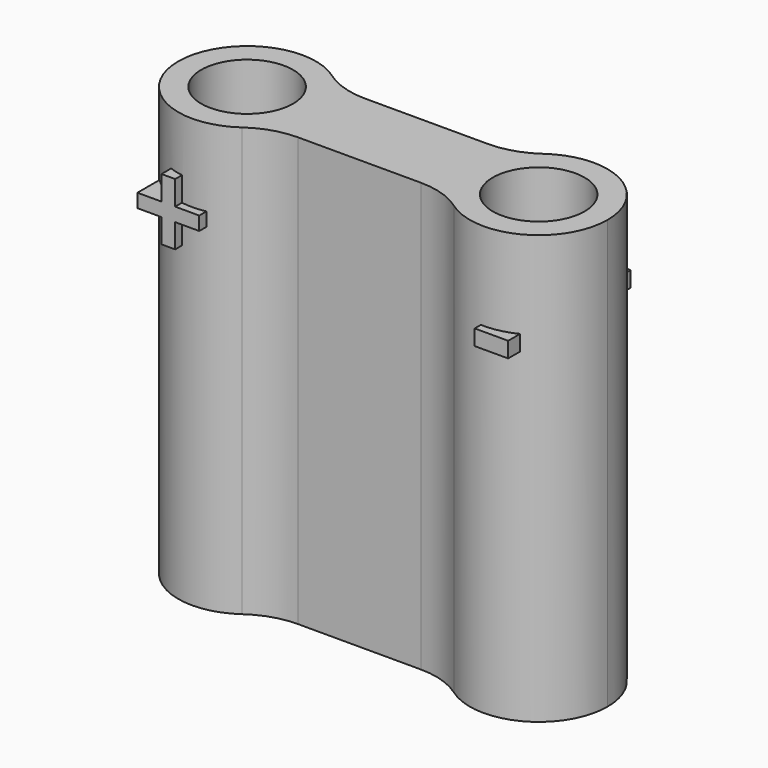
from build123d import *

# Parameters (mm, degrees)
F0_R         = 3
F1_DEPTH     = 28
F2_R         = 5
F3_TEXT_SIZE = 8.3333333333
F4_DEPTH     = 5
F5_DEPTH     = 25


# Not quite as in the source:
# - Text() gives the source's letters only with a copy of the font that has no kerning and outlines rounded to 1/6400 em; it was checked with that copy


with BuildPart() as f1:
    # F0 (on Top) → F1 (new body)
    with BuildSketch(Plane.XY):
        with BuildLine():
            ThreePointArc((-5.9562988107, -2.7412354553), (-5.2641811027, -1.4475573647), (-5.025, 0))
            ThreePointArc((-5.025, 0), (-5.2641811027, 1.4475573647), (-5.9562988107, 2.7412354553))
            ThreePointArc((-5.9562988107, 2.7412354553), (-14.025, 0), (-5.9562988107, -2.7412354553))
        make_face()
        with Locations((-9.525, 0)):
            Circle(F0_R, mode=Mode.SUBTRACT)
        with BuildLine():
            ThreePointArc((-5.9562988107, 2.7412354553), (-5.2641811027, 1.4475573647), (-5.025, 0))
            ThreePointArc((-5.025, 0), (-5.2641811027, -1.4475573647), (-5.9562988107, -2.7412354553))
            Line((-5.9562988107, -2.7412354553), (5.9562988107, -2.7412354553))
            ThreePointArc((5.9562988107, -2.7412354553), (5.025, 0), (5.9562988107, 2.7412354553))
            Line((5.9562988107, 2.7412354553), (-5.9562988107, 2.7412354553))
        make_face()
        with BuildLine():
            ThreePointArc((14.025, 0), (10.9725573647, 4.2608188973), (5.9562988107, 2.7412354553))
            ThreePointArc((5.9562988107, 2.7412354553), (5.025, 0), (5.9562988107, -2.7412354553))
            ThreePointArc((5.9562988107, -2.7412354553), (10.9725573647, -4.2608188973), (14.025, 0))
        make_face()
        with Locations((9.525, 0)):
            Circle(F0_R, mode=Mode.SUBTRACT)
    extrude(amount=F1_DEPTH)

    # F2
    f2_edges = [f1.edges().sort_by_distance(p)[0] for p in [
        (-5.956299, 2.741235, 14),
        (5.956299, 2.741235, 14),
        (5.956299, -2.741235, 14),
        (-5.956299, -2.741235, 14),
    ]]
    fillet(f2_edges, radius=F2_R)

    # F3 (on Front) → F4 (join, symmetric)
    with BuildSketch(Plane.XZ):
        with Locations((-13.0527968763, 19.5263372535)):
            Text('+', F3_TEXT_SIZE, font='Open Sans', font_style=FontStyle.BOLD, text_align=(TextAlign.LEFT, TextAlign.BOTTOM))
        with Locations((9.0964166679, 19.5263372535)):
            Text('-', F3_TEXT_SIZE, font='Open Sans', font_style=FontStyle.BOLD, text_align=(TextAlign.LEFT, TextAlign.BOTTOM))
    extrude(amount=F4_DEPTH, both=True)

    # F0 (on Top) → F5 (cut)
    with BuildSketch(Plane.XY):
        with Locations((9.525, 0)):
            Circle(F0_R)
        with Locations((-9.525, 0)):
            Circle(F0_R)
    extrude(amount=F5_DEPTH, mode=Mode.SUBTRACT)


solid = f1.part
